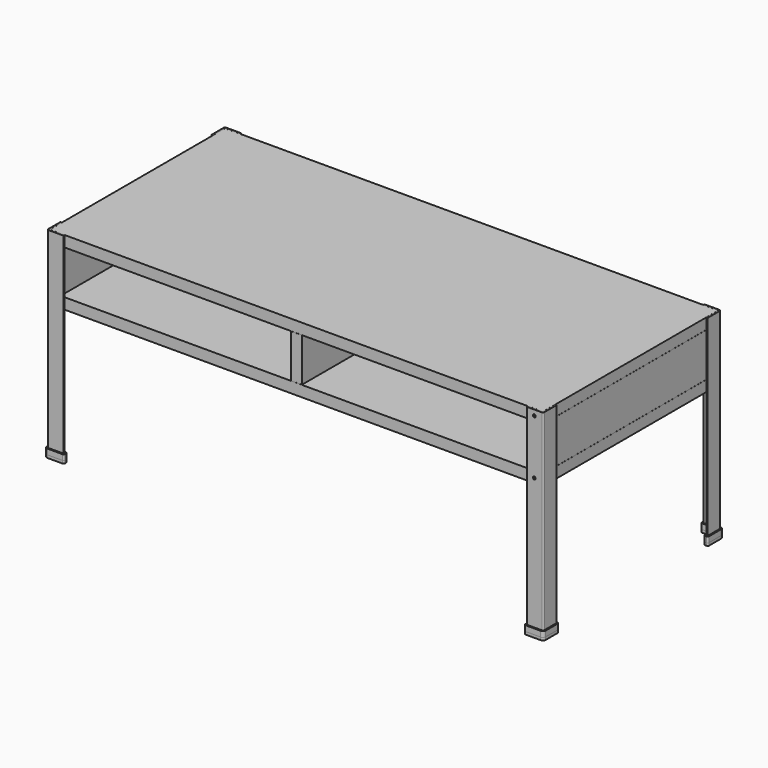
from build123d import *

# Parameters (mm, degrees)
F0_W             = 1143
F0_H             = 508
F1_DEPTH         = 25.4
F2_W             = 25.4
F2_H             = 508
F3_DEPTH         = 101.6
F4_W             = 1143
F4_H             = 508
F5_DEPTH         = 25.4
F6_W             = 25.4
F6_H             = 0.127
F7_DEPTH         = 508.001
F9_DEPTH         = 457.2
F10_R            = 3.175
F10_2_R          = 3.175
F10_3_R          = 3.175
F10_4_R          = 3.175
F11_R            = 3.175
F12_DEPTH        = 3.175
F14_DEPTH        = 12.7
F14_COPIES_COUNT = 2
F15_R            = 3.175
F15_2_R          = 3.175
F17_DEPTH        = 6.35
F23_DEPTH        = 508


# Not quite as in the source:
# - a pattern or mirror of a feature is missing from the dataset's text; its kind, count and spacing are read off the source's solid


with BuildPart() as f1:
    # F0 (on Top) → F1 (new body)
    with BuildSketch(Plane.XY):
        Rectangle(F0_W, F0_H)
    extrude(amount=F1_DEPTH)


with BuildPart() as f3:
    # F2 (on face) → F3 (new body)
    with BuildSketch(Plane.XY.offset(25.4)):
        with Locations((-558.8, 0)):
            Rectangle(F2_W, F2_H)
    extrude(amount=F3_DEPTH)


with BuildPart() as f3b:
    # F2 (on face) → F3, piece 2 (new body)
    with BuildSketch(Plane.XY.offset(25.4)):
        with Locations((558.8, 0)):
            Rectangle(F2_W, F2_H)
    extrude(amount=F3_DEPTH)


with BuildPart() as f5:
    # F4 (on face) → F5 (new body)
    with BuildSketch(Plane.XY.offset(127)):
        Rectangle(F4_W, F4_H)
    extrude(amount=F5_DEPTH)


with BuildPart() as f7_tool:
    # F6 (on face) → F7 (new body, through all)
    with BuildSketch(Plane.XZ.offset(254)):
        with Locations((-558.8, 126.9365)):
            Rectangle(F6_W, F6_H)
        with Locations((558.8, 126.9365)):
            Rectangle(F6_W, F6_H)
        with Locations((-558.8, 25.4635)):
            Rectangle(F6_W, F6_H)
        with Locations((558.8, 25.4635)):
            Rectangle(F6_W, F6_H)
    extrude(amount=-F7_DEPTH)


with BuildPart() as f3_1:
    add(f3.part)

    # F7: cut by f7_tool
    add(f7_tool.part, mode=Mode.SUBTRACT)


with BuildPart() as f3b_1:
    add(f3b.part)

    # F7: cut by f7_tool
    add(f7_tool.part, mode=Mode.SUBTRACT)


with BuildPart() as f9:
    # F8 (on face) → F9 (new body)
    with BuildSketch(Plane.XY.offset(152.4)):
        Polygon((571.627, -254.127), (536.702, -254.127), (536.702, -257.302), (574.802, -257.302), (574.802, -219.202), (571.627, -219.202), align=None)
    extrude(amount=-F9_DEPTH)

    # F10
    f10_edges = [f9.edges().sort_by_distance(p)[0] for p in [
        (574.802, -257.302, -76.2),
    ]]
    fillet(f10_edges, radius=F10_R)

    # F11 (on face) → F12 (cut)
    with BuildSketch(Plane.XZ.offset(257.302)):
        with Locations((554.1645, 139.7)):
            Circle(F11_R)
        with Locations((554.1645, 12.7)):
            Circle(F11_R)
    extrude(amount=-F12_DEPTH, mode=Mode.SUBTRACT)


with BuildPart() as f9b:
    # F8 (on face) → F9, piece 2 (new body)
    with BuildSketch(Plane.XY.offset(152.4)):
        Polygon((571.627, 254.127), (571.627, 219.202), (574.802, 219.202), (574.802, 257.302), (536.702, 257.302), (536.702, 254.127), align=None)
    extrude(amount=-F9_DEPTH)

    # F10#2
    f10_2_edges = [f9b.edges().sort_by_distance(p)[0] for p in [
        (574.802, 257.302, -76.2),
    ]]
    fillet(f10_2_edges, radius=F10_2_R)


with BuildPart() as f9c:
    # F8 (on face) → F9, piece 3 (new body)
    with BuildSketch(Plane.XY.offset(152.4)):
        Polygon((-571.627, -254.127), (-571.627, -219.202), (-574.802, -219.202), (-574.802, -257.302), (-536.702, -257.302), (-536.702, -254.127), align=None)
    extrude(amount=-F9_DEPTH)

    # F10#3
    f10_3_edges = [f9c.edges().sort_by_distance(p)[0] for p in [
        (-574.802, -257.302, -76.2),
    ]]
    fillet(f10_3_edges, radius=F10_3_R)


with BuildPart() as f9d:
    # F8 (on face) → F9, piece 4 (new body)
    with BuildSketch(Plane.XY.offset(152.4)):
        Polygon((-574.802, 257.302), (-574.802, 219.202), (-571.627, 219.202), (-571.627, 254.127), (-536.702, 254.127), (-536.702, 257.302), align=None)
    extrude(amount=-F9_DEPTH)

    # F10#4
    f10_4_edges = [f9d.edges().sort_by_distance(p)[0] for p in [
        (-574.802, 257.302, -76.2),
    ]]
    fillet(f10_4_edges, radius=F10_4_R)


with BuildPart() as f14:
    # F13 (on face) → F14 (new body)
    with BuildSketch(Plane(origin=(0, 0, -304.8), x_dir=(1, 0, 0), z_dir=(0, 0, -1))):
        with BuildLine():
            Line((-533.4, 260.604), (-571.627, 260.604))
            ThreePointArc((-571.627, 260.604), (-576.2069306217, 258.7069306217), (-578.104, 254.127))
            Line((-578.104, 254.127), (-578.104, 215.9))
            Line((-578.104, 215.9), (-568.325, 215.9))
            Line((-568.325, 215.9), (-568.325, 250.825))
            Line((-568.325, 250.825), (-533.4, 250.825))
            Line((-533.4, 250.825), (-533.4, 260.604))
        make_face()
        with BuildLine():
            ThreePointArc((-574.929, 254.127), (-573.9618665915, 256.4618665915), (-571.627, 257.429))
            Line((-571.627, 257.429), (-536.575, 257.429))
            Line((-536.575, 257.429), (-536.575, 254))
            Line((-536.575, 254), (-571.5, 254))
            Line((-571.5, 254), (-571.5, 219.075))
            Line((-571.5, 219.075), (-574.929, 219.075))
            Line((-574.929, 219.075), (-574.929, 254.127))
        make_face(mode=Mode.SUBTRACT)
    extrude(amount=-F14_DEPTH)


with BuildPart() as f14_copies_1:
    # F14_copies: instance of F14
    add(f14.part.rotate(Axis((0, 0, 0), (0, 0, 1)), 1 * 360 / F14_COPIES_COUNT))

    # F15#2
    f15_2_edges = [f14_copies_1.edges().sort_by_distance(p)[0] for p in [
        (533.4, 260.604, -298.45),
        (578.104, 215.9, -298.45),
        (568.325, 215.9, -298.45),
        (533.4, 250.825, -298.45),
    ]]
    fillet(f15_2_edges, radius=F15_2_R)


with BuildPart() as f14_1:
    add(f14.part)

    # F15
    f15_edges = [f14_1.edges().sort_by_distance(p)[0] for p in [
        (-533.4, -260.604, -298.45),
        (-533.4, -250.825, -298.45),
        (-568.325, -215.9, -298.45),
        (-578.104, -215.9, -298.45),
    ]]
    fillet(f15_edges, radius=F15_R)


with BuildPart() as f17:
    # F16 (on face) → F17 (new body)
    with BuildSketch(Plane(origin=(0, 0, -304.8), x_dir=(1, 0, 0), z_dir=(0, 0, -1))):
        with BuildLine():
            Line((-568.325, 250.825), (-536.575, 250.825))
            ThreePointArc((-536.575, 250.825), (-534.3299359697, 251.7549359697), (-533.4, 254))
            Line((-533.4, 254), (-533.4, 257.429))
            ThreePointArc((-533.4, 257.429), (-534.3299359697, 259.6740640303), (-536.575, 260.604))
            Line((-536.575, 260.604), (-571.627, 260.604))
            ThreePointArc((-571.627, 260.604), (-576.2069306217, 258.7069306217), (-578.104, 254.127))
            Line((-578.104, 254.127), (-578.104, 219.075))
            ThreePointArc((-578.104, 219.075), (-577.1740640303, 216.8299359697), (-574.929, 215.9))
            Line((-574.929, 215.9), (-571.5, 215.9))
            ThreePointArc((-571.5, 215.9), (-569.2549359697, 216.8299359697), (-568.325, 219.075))
            Line((-568.325, 219.075), (-568.325, 250.825))
        make_face()
    extrude(amount=F17_DEPTH)


with BuildPart() as f18_1:
    # F18: instance of F14
    add(f14_1.part.mirror(Plane.XZ))


with BuildPart() as f19_1:
    # F19: instance of F14
    add(f14_1.part.mirror(Plane.YZ))


with BuildPart() as f20_1:
    # F20: instance of F17
    add(f17.part.mirror(Plane.YZ))


with BuildPart() as f21_1:
    # F21: instance of F17
    add(f17.part.mirror(Plane.XZ))


with BuildPart() as f21_2:
    # F21: instance of F20_1
    add(f20_1.part.mirror(Plane.XZ))


with BuildPart() as f23:
    # F22 (on face) → F23 (new body, through all)
    with BuildSketch(Plane.XZ.offset(254)):
        Polygon((12.7, 126.873), (0, 126.873), (-12.7, 126.873), (-12.7, 25.527), (0, 25.527), (12.7, 25.527), align=None)
    extrude(amount=-F23_DEPTH)


solid = Compound([f1.part, f5.part, f3_1.part, f3b_1.part, f9.part, f9b.part, f9c.part, f9d.part, f14_copies_1.part, f14_1.part, f17.part, f18_1.part, f19_1.part, f20_1.part, f21_1.part, f21_2.part, f23.part])
